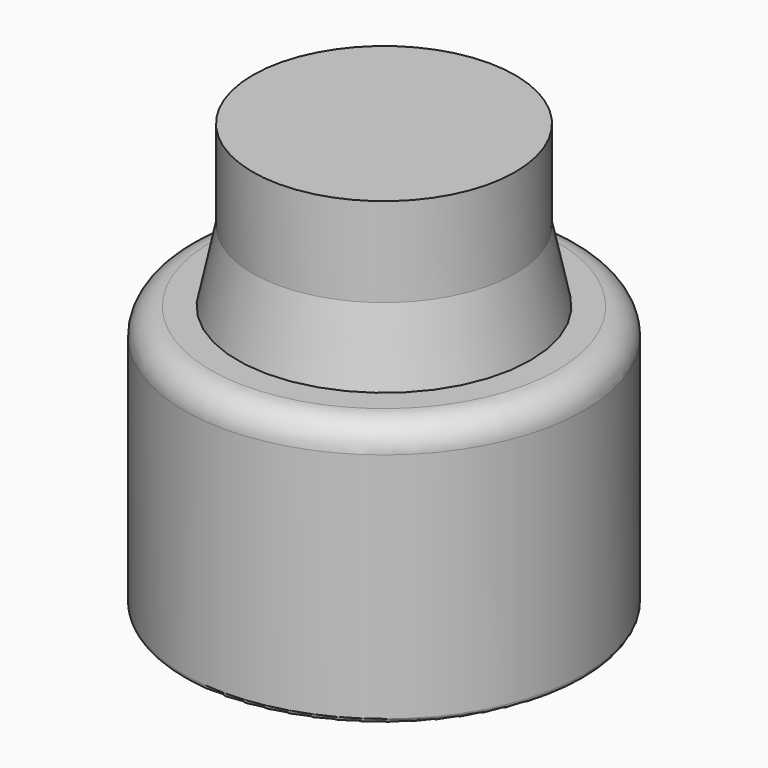
from build123d import *

# Parameters (mm, degrees)
F2_R     = 6.0755158613
F3_DEPTH = 11.8
F4_R     = 5.675
F5_DEPTH = 1
F5_TAPER = 70


# Not quite as in the source:
# - an extrude ends at something that could not be found from the text; its depth is read off the source's solid


with BuildPart() as f1:
    # F0 (on Front) → F1 (revolve)
    with BuildSketch(Plane.XZ):
        with BuildLine():
            Line((7.75, 11.8), (5.675, 11.8))
            Line((5.675, 11.8), (5.675, 6.8))
            Line((5.675, 6.8), (1.5, 4.3895626261))
            Line((1.5, 4.3895626261), (0, 4.3895626261))
            Line((0, 4.3895626261), (0, 0))
            Line((0, 0), (8.75, 0))
            ThreePointArc((8.75, 0), (8.8914213562, 0.0585786438), (8.95, 0.2))
            Line((8.95, 0.2), (8.95, 10.6))
            ThreePointArc((8.95, 10.6), (8.5985281374, 11.4485281374), (7.75, 11.8))
        make_face()
    revolve(axis=Axis((0, 0, 2.1947813131), (0, 0, -1)))

    # F2 (on face) → F3 (join, through all)
    with BuildSketch(Plane.XY.offset(11.8)):
        Circle(F2_R)
        with BuildLine():
            ThreePointArc((-1.0963258128, 4.8337596162), (0, 5.675), (1.0963258128, 4.8337596162))
            Line((1.0963258128, 4.8337596162), (1.1194292397, 4.7475364534))
            ThreePointArc((1.1194292397, 4.7475364534), (2.0447579307, 3.5416246251), (3.5517725542, 3.343222386))
            Line((3.5517725542, 3.343222386), (3.637995717, 3.3663258128))
            ThreePointArc((3.637995717, 3.3663258128), (4.9146941665, 2.8375), (4.7343215298, 1.4674338034))
            Line((4.7343215298, 1.4674338034), (4.6712017939, 1.4043140674))
            ThreePointArc((4.6712017939, 1.4043140674), (4.0895158613, 0), (4.6712017939, -1.4043140674))
            Line((4.6712017939, -1.4043140674), (4.7343215298, -1.4674338034))
            ThreePointArc((4.7343215298, -1.4674338034), (4.9146941665, -2.8375), (3.637995717, -3.3663258128))
            Line((3.637995717, -3.3663258128), (3.5517725542, -3.343222386))
            ThreePointArc((3.5517725542, -3.343222386), (2.0447579307, -3.5416246251), (1.1194292397, -4.7475364534))
            Line((1.1194292397, -4.7475364534), (1.0963258128, -4.8337596162))
            ThreePointArc((1.0963258128, -4.8337596162), (0, -5.675), (-1.0963258128, -4.8337596162))
            Line((-1.0963258128, -4.8337596162), (-1.1194292397, -4.7475364534))
            ThreePointArc((-1.1194292397, -4.7475364534), (-2.0447579307, -3.5416246251), (-3.5517725542, -3.343222386))
            Line((-3.5517725542, -3.343222386), (-3.637995717, -3.3663258128))
            ThreePointArc((-3.637995717, -3.3663258128), (-4.9146941665, -2.8375), (-4.7343215298, -1.4674338034))
            Line((-4.7343215298, -1.4674338034), (-4.6712017939, -1.4043140674))
            ThreePointArc((-4.6712017939, -1.4043140674), (-4.0895158613, 0), (-4.6712017939, 1.4043140674))
            Line((-4.6712017939, 1.4043140674), (-4.7343215298, 1.4674338034))
            ThreePointArc((-4.7343215298, 1.4674338034), (-4.9146941665, 2.8375), (-3.637995717, 3.3663258128))
            Line((-3.637995717, 3.3663258128), (-3.5517725542, 3.343222386))
            ThreePointArc((-3.5517725542, 3.343222386), (-2.0447579307, 3.5416246251), (-1.1194292397, 4.7475364534))
            Line((-1.1194292397, 4.7475364534), (-1.0963258128, 4.8337596162))
        make_face(mode=Mode.SUBTRACT)
    extrude(amount=-F3_DEPTH)

    # F4 (on face) → F5 (cut)
    with BuildSketch(Plane.XY.offset(11.8)):
        Circle(F4_R)
    extrude(amount=-F5_DEPTH, taper=F5_TAPER, mode=Mode.SUBTRACT)


with BuildPart() as f7:
    # F6 (on Front) → F7 (revolve)
    with BuildSketch(Plane.XZ):
        with BuildLine():
            Line((5.875, 19), (0, 19))
            Line((0, 19), (0, 0))
            Line((0, 0), (5.865, 0))
            Line((5.865, 0), (7.0647936412, 6.4735071969))
            ThreePointArc((7.0647936412, 6.4735071969), (7.1980690013, 8.0361081654), (7.0239351866, 9.5946849274))
            Line((7.0239351866, 9.5946849274), (5.875, 15))
            Line((5.875, 15), (5.875, 19))
        make_face()
    revolve(axis=Axis((0, 0, 9.5), (0, 0, -1)))


with BuildPart() as f9:
    # F8 (on Front) → F9 (revolve)
    with BuildSketch(Plane.XZ):
        with BuildLine():
            Line((0, 10.2065285868), (0, 0))
            Line((0, 0), (7.6794893927, 0))
            ThreePointArc((7.6794893927, 0), (8.0188897655, 0.1328387453), (8.1779480596, 0.4607704521))
            Line((8.1779480596, 0.4607704521), (8.8099605555, 8.4912506207))
            ThreePointArc((8.8099605555, 8.4912506207), (8.8334940086, 9.4726497172), (8.75, 10.4507738201))
            ThreePointArc((8.75, 10.4507738201), (8.5926503421, 10.7497954303), (8.2810404532, 10.8804557354))
            Line((8.2810404532, 10.8804557354), (6, 11))
            Line((6, 11), (1.5, 10.2065285868))
            Line((1.5, 10.2065285868), (0, 10.2065285868))
        make_face()
    revolve(axis=Axis((0, 0, 5.1032642934), (0, 0, 1)))


solid = Compound([f1.part, f7.part, f9.part])
